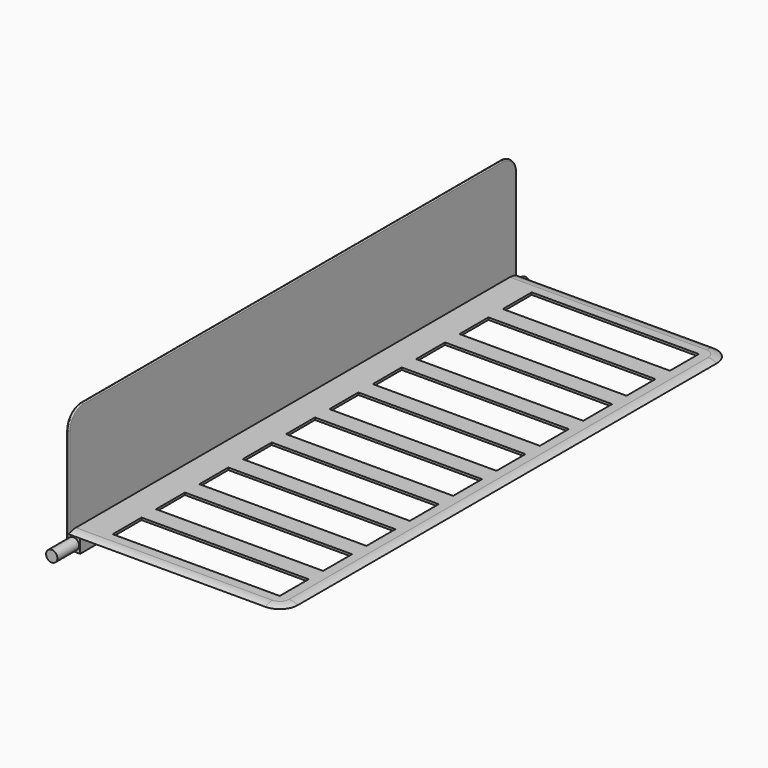
from build123d import *

# Parameters (mm, degrees)
F0_W         = 6.35
F0_H         = 298.45
F0_W_2       = 603.25
F0_H_2       = 6.35
F1_DEPTH     = 1574.8
F2_W         = 38.1
F2_H         = 38.1
F3_DEPTH     = 1574.8
F4_R         = 15.875
F5_DEPTH     = 76.2
F6_R         = 15.875
F7_DEPTH     = 12.7
F8_W         = 469.9
F8_H         = 101.6
F9_DEPTH     = 25.4
F10_R        = 50.8
F11_T1_DEPTH = 1473.2
F11_T3_DEPTH = 552.45
F11_T6_ANGLE = 90
F11_T8_ANGLE = 90
F12_R        = 3.17499


# Not quite as in the source:
# - a fillet or chamfer that OpenCascade refuses, or shapes differently, is made with other operations: its cross-section is extruded or revolved along the edge and cut away or added
# - a fillet or chamfer is up to 0.001 mm smaller than in the source, because OpenCascade refuses the exact size


with BuildPart() as f1:
    # F0 (on Front) → F1 (new body)
    with BuildSketch(Plane.XZ):
        with Locations((3.175, 155.575)):
            Rectangle(F0_W, F0_H)
        with Locations((307.975, 3.175)):
            Rectangle(F0_W_2, F0_H_2)
        with Locations((3.175, 3.175)):
            Rectangle(F0_W, F0_H_2)
    extrude(amount=F1_DEPTH)

    # F2 (on face) → F3 (join)
    with BuildSketch(Plane.XZ.offset(1574.8)):
        with Locations((19.05, -19.05)):
            Rectangle(F2_W, F2_H)
    extrude(amount=-F3_DEPTH)

    # F4 (on face) → F5 (join)
    with BuildSketch(Plane.XZ.offset(1574.8)):
        with Locations((19.05, -19.05)):
            Circle(F4_R)
    extrude(amount=F5_DEPTH)

    # F6 (on face) → F7 (join)
    with BuildSketch(Plane(origin=(0, 0, 0), x_dir=(-1, 0, 0), z_dir=(0, 1, 0))):
        with Locations((-19.05, -19.05)):
            Circle(F6_R)
    extrude(amount=F7_DEPTH)

    # F8 (on face) → F9 (cut)
    with BuildSketch(Plane(origin=(0, 0, 0), x_dir=(1, 0, 0), z_dir=(0, 0, -1))):
        with Locations((323.85, 1473.2)):
            Rectangle(F8_W, F8_H)
        with Locations((323.85, 1320.8)):
            Rectangle(F8_W, F8_H)
        with Locations((323.85, 1168.4)):
            Rectangle(F8_W, F8_H)
        with Locations((323.85, 1016)):
            Rectangle(F8_W, F8_H)
        with Locations((323.85, 863.6)):
            Rectangle(F8_W, F8_H)
        with Locations((323.85, 711.2)):
            Rectangle(F8_W, F8_H)
        with Locations((323.85, 558.8)):
            Rectangle(F8_W, F8_H)
        with Locations((323.85, 406.4)):
            Rectangle(F8_W, F8_H)
        with Locations((323.85, 254)):
            Rectangle(F8_W, F8_H)
        with Locations((323.85, 101.6)):
            Rectangle(F8_W, F8_H)
    extrude(amount=-F9_DEPTH, mode=Mode.SUBTRACT)

    # F10
    f10_edges = [f1.edges().sort_by_distance(p)[0] for p in [
        (609.6, 0, 3.175),
        (609.6, -1574.8, 3.175),
        (3.175, -1574.8, 304.8),
        (3.175, 0, 304.8),
    ]]
    fillet(f10_edges, radius=F10_R)

    # F11: fillet of radius 50.8 on 1 edges, made by hand

    # F11_s2 → F11_t1 (cut)
    with BuildSketch(Plane.XZ.offset(50.8)):
        with BuildLine():
            ThreePointArc((585.0065557516, 6.35), (597.7065557516, 4.7368884968), (609.6, 0))
            Line((609.6, 0), (609.6, 6.35))
            Line((609.6, 6.35), (585.0065557516, 6.35))
        make_face()
    extrude(amount=F11_T1_DEPTH, mode=Mode.SUBTRACT)

    # F11_s4 → F11_t3 (cut)
    with BuildSketch(Plane.YZ.offset(6.35)):
        with BuildLine():
            ThreePointArc((-1574.8, 0), (-1562.9065557516, 4.7368884968), (-1550.2065557516, 6.35))
            Line((-1550.2065557516, 6.35), (-1574.8, 6.35))
            Line((-1574.8, 6.35), (-1574.8, 0))
        make_face()
        with BuildLine():
            ThreePointArc((0, 0), (-11.8934442484, 4.7368884968), (-24.5934442484, 6.35))
            Line((-24.5934442484, 6.35), (0, 6.35))
            Line((0, 6.35), (0, 0))
        make_face()
    extrude(amount=F11_T3_DEPTH, mode=Mode.SUBTRACT)

    # F11_s5 → F11_t6 (revolve, cut)
    with BuildSketch(Plane.YZ.offset(558.8)):
        with BuildLine():
            ThreePointArc((-24.5934442484, 6.35), (-11.8934442484, 4.7368884968), (0, 0))
            Line((0, 0), (0, 6.35))
            Line((0, 6.35), (-24.5934442484, 6.35))
        make_face()
    revolve(axis=Axis((558.8, -50.8, 6.35), (0, 0, -1)), revolution_arc=F11_T6_ANGLE, mode=Mode.SUBTRACT)

    # F11_s7 → F11_t8 (revolve, cut)
    with BuildSketch(Plane.YZ.offset(558.8)):
        with BuildLine():
            ThreePointArc((-1550.2065557516, 6.35), (-1562.9065557516, 4.7368884968), (-1574.8, 0))
            Line((-1574.8, 0), (-1574.8, 6.35))
            Line((-1574.8, 6.35), (-1550.2065557516, 6.35))
        make_face()
    revolve(axis=Axis((558.8, -1524, 6.35), (0, 0, 1)), revolution_arc=F11_T8_ANGLE, mode=Mode.SUBTRACT)

    # F12 (radius 3.175 in the source; OpenCascade refuses exactly that, so slightly less here)
    f12_edges = [f1.edges().sort_by_distance(p)[0] for p in [
        (6.35, -787.4, 304.8),
        (0, -787.4, 304.8),
        (0, -14.878976, 289.921024),
        (0, -1559.921024, 289.921024),
        (0, 0, 107.95),
        (0, -1574.8, 107.95),
        (6.35, -14.878976, 289.921024),
        (6.35, -1559.921024, 289.921024),
        (6.35, 0, 127),
        (6.35, -1574.8, 127),
    ]]
    fillet(f12_edges, radius=F12_R)


solid = f1.part
